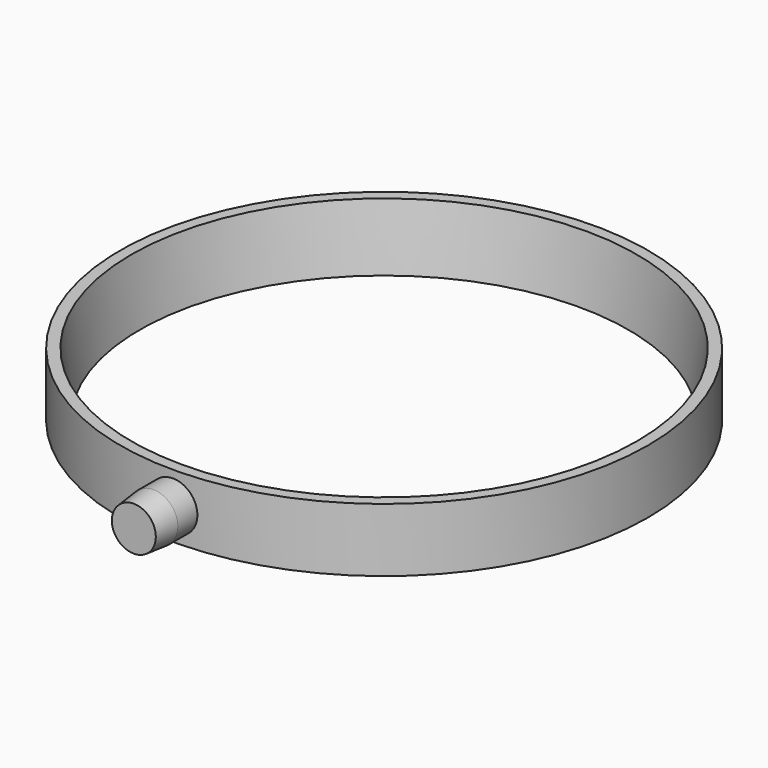
from build123d import *

# Parameters (mm, degrees)
F0_R     = 54
F0_R_2   = 50
F1_DEPTH = 13
F3_R     = 5
F4_DEPTH = 10
F5_SIZE2 = 1.711472
F5_SIZE  = 12.99999
F6_SIZE2 = 5
F6_SIZE  = 0.5


# Not quite as in the source:
# - a fillet or chamfer is up to 0.001 mm smaller than in the source, because OpenCascade refuses the exact size


with BuildPart() as f1:
    # F0 (on Top) → F1 (new body)
    with BuildSketch(Plane.XY):
        Circle(F0_R)
        Circle(F0_R_2, mode=Mode.SUBTRACT)
    extrude(amount=F1_DEPTH)

    # F3 (on offset) → F4 (join)
    with BuildSketch(Plane.XZ.offset(54)):
        with Locations((0, 6.4556576599)):
            Circle(F3_R)
    extrude(amount=F4_DEPTH)

    # F5 (size 13 and 1.7114824686 in the source; OpenCascade refuses exactly that, so slightly less here)
    f5_edges = [f1.edges().sort_by_distance(p)[0] for p in [
        (-50, 0, 13),
    ]]
    f5_side = f1.faces().sort_by_distance((-50, 0, 6.5))[0]
    chamfer(f5_edges, length=F5_SIZE, length2=F5_SIZE2, reference=f5_side)

    # F6
    f6_edges = [f1.edges().sort_by_distance(p)[0] for p in [
        (-5, -64, 6.455658),
    ]]
    f6_side = f1.faces().sort_by_distance((0, -64, 6.455658))[0]
    chamfer(f6_edges, length=F6_SIZE, length2=F6_SIZE2, reference=f6_side)


solid = f1.part
